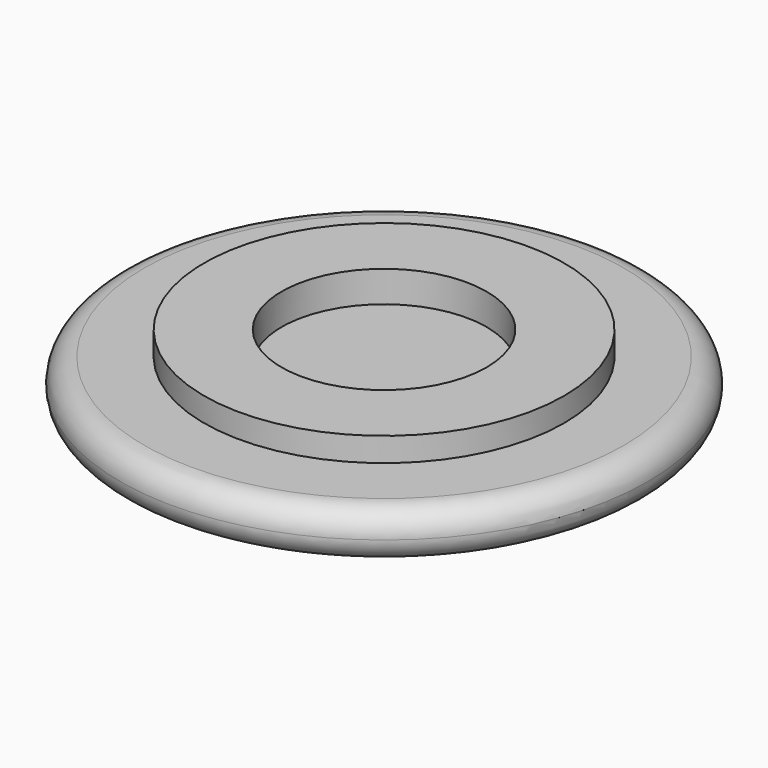
from build123d import *

# Parameters (mm, degrees)
F0_R     = 11
F0_R_2   = 7.5
F1_DEPTH = 2
F0_R_3   = 4.275
F2_DEPTH = 3
F3_DEPTH = 1.7
F4_R     = 0.99999


# Not quite as in the source:
# - a fillet or chamfer is up to 0.001 mm smaller than in the source, because OpenCascade refuses the exact size


with BuildPart() as f1:
    # F0 (on Top) → F1 (new body)
    with BuildSketch(Plane.XY):
        Circle(F0_R)
        Circle(F0_R_2, mode=Mode.SUBTRACT)
    extrude(amount=F1_DEPTH)

    # F0 (on Top) → F2 (join)
    with BuildSketch(Plane.XY):
        Circle(F0_R_2)
        Circle(F0_R_3, mode=Mode.SUBTRACT)
    extrude(amount=F2_DEPTH)

    # F0 (on Top) → F3 (join)
    with BuildSketch(Plane.XY):
        Circle(F0_R_3)
    extrude(amount=F3_DEPTH)

    # F4 (radius 1 in the source; OpenCascade refuses exactly that, so slightly less here)
    f4_edges = [f1.edges().sort_by_distance(p)[0] for p in [
        (-11, 0, 2),
        (-11, 0, 0),
    ]]
    fillet(f4_edges, radius=F4_R)


solid = f1.part
